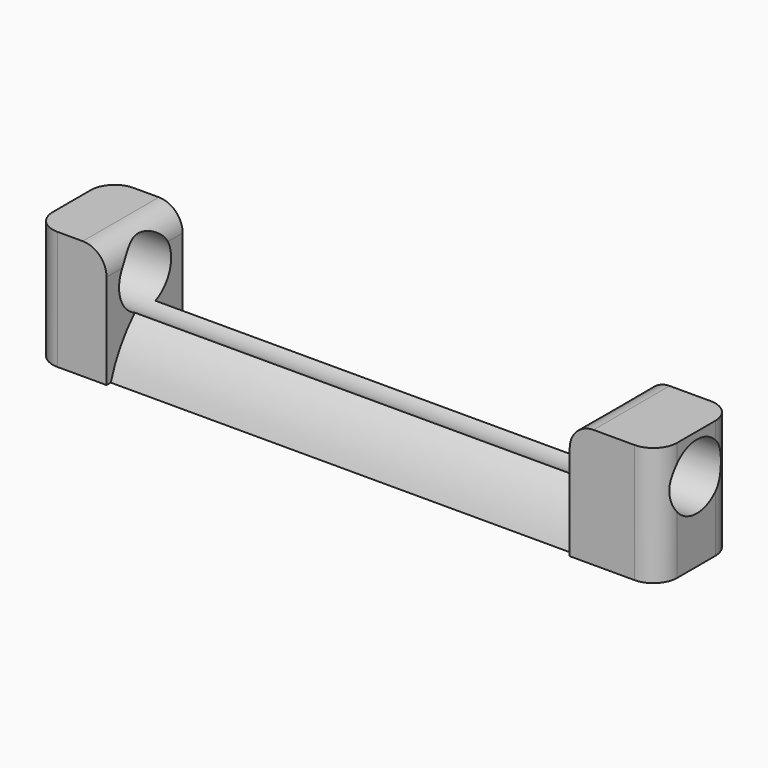
from build123d import *

# Parameters (mm, degrees)
F0_W         = 26.2500010431
F0_H         = 4
F1_DEPTH     = 5
F2_W         = 19.4687498733
F2_H         = 4.5937502291
F3_DEPTH     = 43.3
F4_DEPTH     = 52.6
F5_R         = 1.3682808459
F6_DEPTH     = 25
F7_DEPTH     = 21.1
F8_T1_DEPTH  = 10
F9_T1_DEPTH  = 10
F10_T1_DEPTH = 10
F11_T1_DEPTH = 19.4687498733
F12_T1_DEPTH = 9


# Not quite as in the source:
# - a fillet or chamfer that OpenCascade refuses, or shapes differently, is made with other operations: its cross-section is extruded or revolved along the edge and cut away or added


with BuildPart() as f1:
    # F0 (on Top) → F1 (new body)
    with BuildSketch(Plane.XY):
        with Locations((-1.4218753204, -1.8281253073)):
            Rectangle(F0_W, F0_H)
    extrude(amount=F1_DEPTH)

    # F2 (on Front) → F3 (cut)
    with BuildSketch(Plane.XZ):
        with Locations((-1.7500002868, 4.375000135)):
            Rectangle(F2_W, F2_H)
    extrude(amount=F3_DEPTH, mode=Mode.SUBTRACT)

    # F2 (on Front) → F4 (cut)
    with BuildSketch(Plane.XZ):
        with Locations((-1.7500002868, 4.375000135)):
            Rectangle(F2_W, F2_H)
    extrude(amount=-F4_DEPTH, mode=Mode.SUBTRACT)

    # F5 (on Right) → F6 (cut)
    with BuildSketch(Plane.YZ):
        with Locations((-1.802527695, 3.3346994314)):
            Circle(F5_R)
    extrude(amount=-F6_DEPTH, mode=Mode.SUBTRACT)

    # F5 (on Right) → F7 (cut)
    with BuildSketch(Plane.YZ):
        with Locations((-1.802527695, 3.3346994314)):
            Circle(F5_R)
    extrude(amount=F7_DEPTH, mode=Mode.SUBTRACT)

    # F8: fillet of radius 1 on 1 edges, made by hand

    # F8_s2 → F8_t1 (cut)
    with BuildSketch(Plane.XY.offset(-2.5)):
        with BuildLine():
            ThreePointArc((10.7031252012, 0.1718746927), (11.4102319824, -0.1210185261), (11.7031252012, -0.8281253073))
            Line((11.7031252012, -0.8281253073), (11.7031252012, 0.1718746927))
            Line((11.7031252012, 0.1718746927), (10.7031252012, 0.1718746927))
        make_face()
    extrude(amount=F8_T1_DEPTH, mode=Mode.SUBTRACT)

    # F9: fillet of radius 1 on 1 edges, made by hand

    # F9_s2 → F9_t1 (cut)
    with BuildSketch(Plane.XY.offset(-2.5)):
        with BuildLine():
            ThreePointArc((-13.5468758419, 0.1718746927), (-14.2539826231, -0.1210185261), (-14.5468758419, -0.8281253073))
            Line((-14.5468758419, -0.8281253073), (-14.5468758419, 0.1718746927))
            Line((-14.5468758419, 0.1718746927), (-13.5468758419, 0.1718746927))
        make_face()
    extrude(amount=F9_T1_DEPTH, mode=Mode.SUBTRACT)

    # F10: fillet of radius 1 on 2 edges, made by hand

    # F10_s2 → F10_t1 (cut)
    with BuildSketch(Plane.XY.offset(-2.5)):
        with BuildLine():
            ThreePointArc((11.7031252012, -2.8281253073), (11.4102319824, -3.5352320885), (10.7031252012, -3.8281253073))
            Line((10.7031252012, -3.8281253073), (11.7031252012, -3.8281253073))
            Line((11.7031252012, -3.8281253073), (11.7031252012, -2.8281253073))
        make_face()
        with BuildLine():
            ThreePointArc((-13.5468758419, -3.8281253073), (-14.2539826231, -3.5352320885), (-14.5468758419, -2.8281253073))
            Line((-14.5468758419, -2.8281253073), (-14.5468758419, -3.8281253073))
            Line((-14.5468758419, -3.8281253073), (-13.5468758419, -3.8281253073))
        make_face()
    extrude(amount=F10_T1_DEPTH, mode=Mode.SUBTRACT)

    # F11: fillet of radius 5 on 2 edges, made by hand

    # F11_s2 → F11_t1 (cut)
    with BuildSketch(Plane.YZ.offset(-11.4843752235)):
        with BuildLine():
            ThreePointArc((0.1718746927, -1.4255693283), (-0.2001967002, 0.467121034), (-1.2610360303, 2.0781250205))
            Line((-1.2610360303, 2.0781250205), (0.1718746927, 2.0781250205))
            Line((0.1718746927, 2.0781250205), (0.1718746927, -1.4255693283))
        make_face()
        with BuildLine():
            ThreePointArc((-3.8281253073, -1.4769402409), (-3.4422054032, 0.4492645429), (-2.3440193596, 2.0781250205))
            Line((-2.3440193596, 2.0781250205), (-3.8281253073, 2.0781250205))
            Line((-3.8281253073, 2.0781250205), (-3.8281253073, -1.4769402409))
        make_face()
    extrude(amount=F11_T1_DEPTH, mode=Mode.SUBTRACT)

    # F12: fillet of radius 1 on 2 edges, made by hand

    # F12_s2 → F12_t1 (cut)
    with BuildSketch(Plane.XZ.offset(-2.6718746927)):
        with BuildLine():
            ThreePointArc((7.9843746498, 4), (8.2772678686, 4.7071067812), (8.9843746498, 5))
            Line((8.9843746498, 5), (7.9843746498, 5))
            Line((7.9843746498, 5), (7.9843746498, 4))
        make_face()
        with BuildLine():
            ThreePointArc((-11.4843752235, 4), (-11.7772684423, 4.7071067812), (-12.4843752235, 5))
            Line((-12.4843752235, 5), (-11.4843752235, 5))
            Line((-11.4843752235, 5), (-11.4843752235, 4))
        make_face()
    extrude(amount=F12_T1_DEPTH, mode=Mode.SUBTRACT)


solid = f1.part
